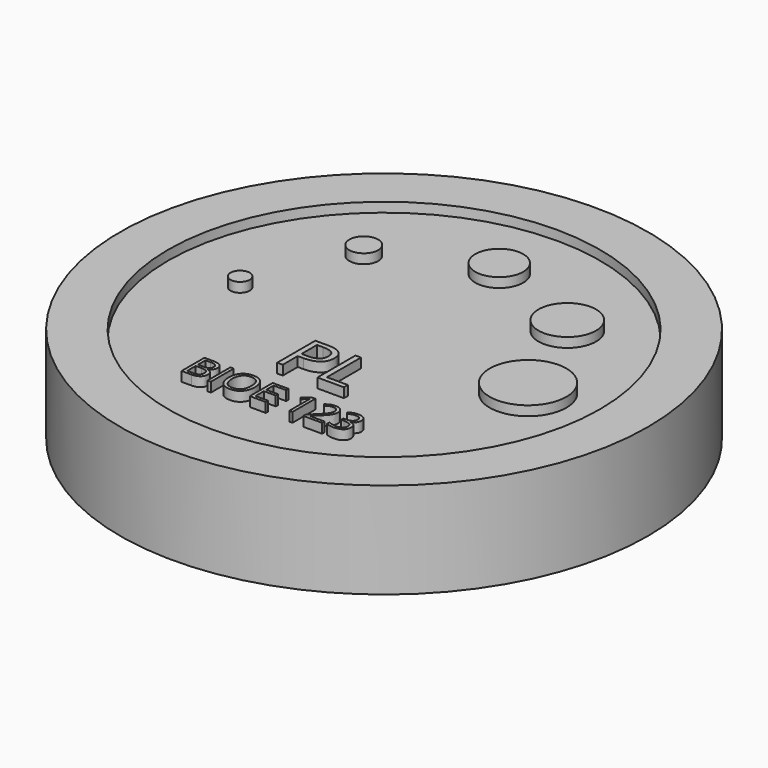
from build123d import *

# Parameters (mm, degrees)
F0_R           = 27.5
F0_R_2         = 22.5
F0_R_3         = 4
F0_R_4         = 3
F0_R_5         = 2.5
F0_R_6         = 1.5
F0_TEXT_SIZE   = 6.9444444444
F0_R_7         = 1
F0_TEXT_SIZE_2 = 4.1666666667
F1_DEPTH       = 10
F0_W           = 0.345703125
F0_H           = 2.974609375
F2_DEPTH       = 3
F4_R           = 22.5
F4_W           = 0.345703125
F4_H           = 2.974609375
F4_R_2         = 1
F4_R_3         = 1.5
F4_R_4         = 3
F4_R_5         = 4
F4_R_6         = 2.5
F5_DEPTH       = 6


# Not quite as in the source:
# - Text() gives the source's letters only with a copy of the font that has no kerning and outlines rounded to 1/6400 em; it was checked with that copy


with BuildPart() as f1:
    # F0 (on Top) → F1 (new body)
    with BuildSketch(Plane.XY):
        Circle(F0_R)
        Circle(F0_R_2, mode=Mode.SUBTRACT)
        with Locations((15, 0)):
            Circle(F0_R_3)
        with Locations((10.6032023465, 10.61)):
            Circle(F0_R_4)
        with Locations((0, 15)):
            Circle(F0_R_5)
        with Locations((-10.6032023465, 10.61)):
            Circle(F0_R_6)
        with Locations((-3.8129340278, -10)):
            Text('PL', F0_TEXT_SIZE, font='Open Sans', text_align=(TextAlign.LEFT, TextAlign.BOTTOM))
        with Locations((-15, 0)):
            Circle(F0_R_7)
        with Locations((-8.7041015625, -16)):
            Text('BIOE 123', F0_TEXT_SIZE_2, font='Open Sans', text_align=(TextAlign.LEFT, TextAlign.BOTTOM))
    extrude(amount=F1_DEPTH)


with BuildPart() as f2:
    # F0 (on Top) → F2 (new body)
    with BuildSketch(Plane.XY):
        Circle(F0_R_2)
        with BuildLine():
            Line((-8.2952473958, -16), (-8.2952473958, -13.025390625))
            Line((-8.2952473958, -13.025390625), (-7.4547526042, -13.025390625))
            add(Edge.make_bspline(
                [(-7.4547526042, -13.025390625), (-6.8629557292, -13.025390625), (-6.5983072917, -13.2024739583)],
                knots=[0, 0, 0, 1, 1, 1], degree=2))
            add(Edge.make_bspline(
                [(-6.5983072917, -13.2024739583), (-6.3336588542, -13.3795572917), (-6.3336588542, -13.76171875)],
                knots=[0, 0, 0, 1, 1, 1], degree=2))
            add(Edge.make_bspline(
                [(-6.3336588542, -13.76171875), (-6.3336588542, -14.0266927083), (-6.4811197917, -14.1985677083)],
                knots=[0, 0, 0, 1, 1, 1], degree=2))
            add(Edge.make_bspline(
                [(-6.4811197917, -14.1985677083), (-6.6285807292, -14.3704427083), (-6.9117838542, -14.4212239583)],
                knots=[0, 0, 0, 1, 1, 1], degree=2))
            Line((-6.9117838542, -14.4212239583), (-6.9117838542, -14.44140625))
            add(Edge.make_bspline(
                [(-6.9117838542, -14.44140625), (-6.2340494792, -14.5572916667), (-6.2340494792, -15.1536458333)],
                knots=[0, 0, 0, 1, 1, 1], degree=2))
            add(Edge.make_bspline(
                [(-6.2340494792, -15.1536458333), (-6.2340494792, -15.5520833333), (-6.5035807292, -15.7760416667)],
                knots=[0, 0, 0, 1, 1, 1], degree=2))
            add(Edge.make_bspline(
                [(-6.5035807292, -15.7760416667), (-6.7731119792, -16), (-7.2574869792, -16)],
                knots=[0, 0, 0, 1, 1, 1], degree=2))
            Line((-7.2574869792, -16), (-8.2952473958, -16))
        make_face(mode=Mode.SUBTRACT)
        with Locations((-5.4225260417, -14.5126953125)):
            Rectangle(F0_W, F0_H, mode=Mode.SUBTRACT)
        with BuildLine():
            add(Edge.make_bspline(
                [(-2.2119140625, -13.3854166667), (-1.8518880208, -13.7923177083), (-1.8518880208, -14.5084635417)],
                knots=[0, 0, 0, 1, 1, 1], degree=2))
            add(Edge.make_bspline(
                [(-1.8518880208, -14.5084635417), (-1.8518880208, -15.22265625), (-2.2132161458, -15.6318359375)],
                knots=[0, 0, 0, 1, 1, 1], degree=2))
            add(Edge.make_bspline(
                [(-2.2132161458, -15.6318359375), (-2.5745442708, -16.041015625), (-3.2171223958, -16.041015625)],
                knots=[0, 0, 0, 1, 1, 1], degree=2))
            add(Edge.make_bspline(
                [(-3.2171223958, -16.041015625), (-3.8740234375, -16.041015625), (-4.2311197917, -15.6389973958)],
                knots=[0, 0, 0, 1, 1, 1], degree=2))
            add(Edge.make_bspline(
                [(-4.2311197917, -15.6389973958), (-4.5882161458, -15.2369791667), (-4.5882161458, -14.5045572917)],
                knots=[0, 0, 0, 1, 1, 1], degree=2))
            add(Edge.make_bspline(
                [(-4.5882161458, -14.5045572917), (-4.5882161458, -13.7779947917), (-4.2301432292, -13.3782552083)],
                knots=[0, 0, 0, 1, 1, 1], degree=2))
            add(Edge.make_bspline(
                [(-4.2301432292, -13.3782552083), (-3.8720703125, -12.978515625), (-3.2132161458, -12.978515625)],
                knots=[0, 0, 0, 1, 1, 1], degree=2))
            add(Edge.make_bspline(
                [(-3.2132161458, -12.978515625), (-2.5719401042, -12.978515625), (-2.2119140625, -13.3854166667)],
                knots=[0, 0, 0, 1, 1, 1], degree=2))
        make_face(mode=Mode.SUBTRACT)
        Polygon((0.4690755208, -15.6907552083), (0.4690755208, -16), (-1.1891276042, -16), (-1.1891276042, -13.025390625), (0.4690755208, -13.025390625), (0.4690755208, -13.3326822917), (-0.8434244792, -13.3326822917), (-0.8434244792, -14.291015625), (0.3896484375, -14.291015625), (0.3896484375, -14.5963541667), (-0.8434244792, -14.5963541667), (-0.8434244792, -15.6907552083), align=None, mode=Mode.SUBTRACT)
        with BuildLine():
            add(Edge.make_bspline(
                [(-1.845703125, -5.0423177083), (0.0119357639, -5.0423177083), (0.0119357639, -6.4865451389)],
                knots=[0, 0, 0, 1, 1, 1], degree=2))
            add(Edge.make_bspline(
                [(0.0119357639, -6.4865451389), (0.0119357639, -7.2395833333), (-0.5018446181, -7.6448567708)],
                knots=[0, 0, 0, 1, 1, 1], degree=2))
            add(Edge.make_bspline(
                [(-0.5018446181, -7.6448567708), (-1.015625, -8.0501302083), (-1.9715711806, -8.0501302083)],
                knots=[0, 0, 0, 1, 1, 1], degree=2))
            Line((-1.9715711806, -8.0501302083), (-2.5553385417, -8.0501302083))
            Line((-2.5553385417, -8.0501302083), (-2.5553385417, -10))
            Line((-2.5553385417, -10), (-3.1315104167, -10))
            Line((-3.1315104167, -10), (-3.1315104167, -5.0423177083))
            Line((-3.1315104167, -5.0423177083), (-1.845703125, -5.0423177083))
        make_face(mode=Mode.SUBTRACT)
        with BuildLine():
            Line((3.2561848958, -13.025390625), (3.2561848958, -16))
            Line((3.2561848958, -16), (2.9267578125, -16))
            Line((2.9267578125, -16), (2.9267578125, -13.8802083333))
            add(Edge.make_bspline(
                [(2.9267578125, -13.8802083333), (2.9267578125, -13.615234375), (2.9430338542, -13.3795572917)],
                knots=[0, 0, 0, 1, 1, 1], degree=2))
            add(Edge.make_bspline(
                [(2.9430338542, -13.3795572917), (2.9007161458, -13.4225260417), (2.84765625, -13.4690755208)],
                knots=[0, 0, 0, 1, 1, 1], degree=2))
            add(Edge.make_bspline(
                [(2.84765625, -13.4690755208), (2.7945963542, -13.515625), (2.3636067708, -13.8658854167)],
                knots=[0, 0, 0, 1, 1, 1], degree=2))
            Line((2.3636067708, -13.8658854167), (2.1845703125, -13.6341145833))
            Line((2.1845703125, -13.6341145833), (2.9716796875, -13.025390625))
            Line((2.9716796875, -13.025390625), (3.2561848958, -13.025390625))
        make_face(mode=Mode.SUBTRACT)
        with BuildLine():
            Line((6.3427734375, -15.6868489583), (6.3427734375, -16))
            Line((6.3427734375, -16), (4.3876953125, -16))
            Line((4.3876953125, -16), (4.3876953125, -15.708984375))
            Line((4.3876953125, -15.708984375), (5.1708984375, -14.921875))
            add(Edge.make_bspline(
                [(5.1708984375, -14.921875), (5.5289713542, -14.5592447917), (5.6429036458, -14.4046223958)],
                knots=[0, 0, 0, 1, 1, 1], degree=2))
            add(Edge.make_bspline(
                [(5.6429036458, -14.4046223958), (5.7568359375, -14.25), (5.8138020833, -14.103515625)],
                knots=[0, 0, 0, 1, 1, 1], degree=2))
            add(Edge.make_bspline(
                [(5.8138020833, -14.103515625), (5.8707682292, -13.95703125), (5.8707682292, -13.7884114583)],
                knots=[0, 0, 0, 1, 1, 1], degree=2))
            add(Edge.make_bspline(
                [(5.8707682292, -13.7884114583), (5.8707682292, -13.5501302083), (5.7262369792, -13.4108072917)],
                knots=[0, 0, 0, 1, 1, 1], degree=2))
            add(Edge.make_bspline(
                [(5.7262369792, -13.4108072917), (5.5817057292, -13.271484375), (5.3251953125, -13.271484375)],
                knots=[0, 0, 0, 1, 1, 1], degree=2))
            add(Edge.make_bspline(
                [(5.3251953125, -13.271484375), (5.1402994792, -13.271484375), (4.9742838542, -13.3326822917)],
                knots=[0, 0, 0, 1, 1, 1], degree=2))
            add(Edge.make_bspline(
                [(4.9742838542, -13.3326822917), (4.8082682292, -13.3938802083), (4.6051432292, -13.5546875)],
                knots=[0, 0, 0, 1, 1, 1], degree=2))
            Line((4.6051432292, -13.5546875), (4.4261067708, -13.3248697917))
            add(Edge.make_bspline(
                [(4.4261067708, -13.3248697917), (4.8369140625, -12.9830729167), (5.3212890625, -12.9830729167)],
                knots=[0, 0, 0, 1, 1, 1], degree=2))
            add(Edge.make_bspline(
                [(5.3212890625, -12.9830729167), (5.7405598958, -12.9830729167), (5.978515625, -13.1975911458)],
                knots=[0, 0, 0, 1, 1, 1], degree=2))
            add(Edge.make_bspline(
                [(5.978515625, -13.1975911458), (6.2164713542, -13.412109375), (6.2164713542, -13.7740885417)],
                knots=[0, 0, 0, 1, 1, 1], degree=2))
            add(Edge.make_bspline(
                [(6.2164713542, -13.7740885417), (6.2164713542, -14.0572916667), (6.0576171875, -14.333984375)],
                knots=[0, 0, 0, 1, 1, 1], degree=2))
            add(Edge.make_bspline(
                [(6.0576171875, -14.333984375), (5.8987630208, -14.6106770833), (5.4638671875, -15.0338541667)],
                knots=[0, 0, 0, 1, 1, 1], degree=2))
            Line((5.4638671875, -15.0338541667), (4.8128255208, -15.6705729167))
            Line((4.8128255208, -15.6705729167), (4.8128255208, -15.6868489583))
            Line((4.8128255208, -15.6868489583), (6.3427734375, -15.6868489583))
        make_face(mode=Mode.SUBTRACT)
        with BuildLine():
            add(Edge.make_bspline(
                [(8.3727213542, -13.1813151042), (8.6129557292, -13.3795572917), (8.6129557292, -13.7252604167)],
                knots=[0, 0, 0, 1, 1, 1], degree=2))
            add(Edge.make_bspline(
                [(8.6129557292, -13.7252604167), (8.6129557292, -14.0104166667), (8.453125, -14.19140625)],
                knots=[0, 0, 0, 1, 1, 1], degree=2))
            add(Edge.make_bspline(
                [(8.453125, -14.19140625), (8.2932942708, -14.3723958333), (8.0003255208, -14.43359375)],
                knots=[0, 0, 0, 1, 1, 1], degree=2))
            Line((8.0003255208, -14.43359375), (8.0003255208, -14.4498697917))
            add(Edge.make_bspline(
                [(8.0003255208, -14.4498697917), (8.3583984375, -14.494140625), (8.53125, -14.6774088542)],
                knots=[0, 0, 0, 1, 1, 1], degree=2))
            add(Edge.make_bspline(
                [(8.53125, -14.6774088542), (8.7041015625, -14.8606770833), (8.7041015625, -15.1575520833)],
                knots=[0, 0, 0, 1, 1, 1], degree=2))
            add(Edge.make_bspline(
                [(8.7041015625, -15.1575520833), (8.7041015625, -15.5826822917), (8.4091796875, -15.8118489583)],
                knots=[0, 0, 0, 1, 1, 1], degree=2))
            add(Edge.make_bspline(
                [(8.4091796875, -15.8118489583), (8.1142578125, -16.041015625), (7.5712890625, -16.041015625)],
                knots=[0, 0, 0, 1, 1, 1], degree=2))
            add(Edge.make_bspline(
                [(7.5712890625, -16.041015625), (7.3349609375, -16.041015625), (7.138671875, -16.0052083333)],
                knots=[0, 0, 0, 1, 1, 1], degree=2))
            add(Edge.make_bspline(
                [(7.138671875, -16.0052083333), (6.9423828125, -15.9694010417), (6.7574869792, -15.8802083333)],
                knots=[0, 0, 0, 1, 1, 1], degree=2))
            Line((6.7574869792, -15.8802083333), (6.7574869792, -15.55859375))
            add(Edge.make_bspline(
                [(6.7574869792, -15.55859375), (6.9508463542, -15.654296875), (7.1695963542, -15.7041015625)],
                knots=[0, 0, 0, 1, 1, 1], degree=2))
            add(Edge.make_bspline(
                [(7.1695963542, -15.7041015625), (7.3883463542, -15.75390625), (7.5836588542, -15.75390625)],
                knots=[0, 0, 0, 1, 1, 1], degree=2))
            add(Edge.make_bspline(
                [(7.5836588542, -15.75390625), (8.3544921875, -15.75390625), (8.3544921875, -15.1497395833)],
                knots=[0, 0, 0, 1, 1, 1], degree=2))
            add(Edge.make_bspline(
                [(8.3544921875, -15.1497395833), (8.3544921875, -14.6080729167), (7.5042317708, -14.6080729167)],
                knots=[0, 0, 0, 1, 1, 1], degree=2))
            Line((7.5042317708, -14.6080729167), (7.2112630208, -14.6080729167))
            Line((7.2112630208, -14.6080729167), (7.2112630208, -14.3177083333))
            Line((7.2112630208, -14.3177083333), (7.5081380208, -14.3177083333))
            add(Edge.make_bspline(
                [(7.5081380208, -14.3177083333), (7.8557942708, -14.3177083333), (8.0592447917, -14.1640625)],
                knots=[0, 0, 0, 1, 1, 1], degree=2))
            add(Edge.make_bspline(
                [(8.0592447917, -14.1640625), (8.2626953125, -14.0104166667), (8.2626953125, -13.7376302083)],
                knots=[0, 0, 0, 1, 1, 1], degree=2))
            add(Edge.make_bspline(
                [(8.2626953125, -13.7376302083), (8.2626953125, -13.5201822917), (8.11328125, -13.3958333333)],
                knots=[0, 0, 0, 1, 1, 1], degree=2))
            add(Edge.make_bspline(
                [(8.11328125, -13.3958333333), (7.9638671875, -13.271484375), (7.7073567708, -13.271484375)],
                knots=[0, 0, 0, 1, 1, 1], degree=2))
            add(Edge.make_bspline(
                [(7.7073567708, -13.271484375), (7.5120442708, -13.271484375), (7.3391927083, -13.3245442708)],
                knots=[0, 0, 0, 1, 1, 1], degree=2))
            add(Edge.make_bspline(
                [(7.3391927083, -13.3245442708), (7.1663411458, -13.3776041667), (6.9443359375, -13.5201822917)],
                knots=[0, 0, 0, 1, 1, 1], degree=2))
            Line((6.9443359375, -13.5201822917), (6.7737630208, -13.2923177083))
            add(Edge.make_bspline(
                [(6.7737630208, -13.2923177083), (6.9567057292, -13.1477864583), (7.1956380208, -13.0654296875)],
                knots=[0, 0, 0, 1, 1, 1], degree=2))
            add(Edge.make_bspline(
                [(7.1956380208, -13.0654296875), (7.4345703125, -12.9830729167), (7.6995442708, -12.9830729167)],
                knots=[0, 0, 0, 1, 1, 1], degree=2))
            add(Edge.make_bspline(
                [(7.6995442708, -12.9830729167), (8.1324869792, -12.9830729167), (8.3727213542, -13.1813151042)],
                knots=[0, 0, 0, 1, 1, 1], degree=2))
        make_face(mode=Mode.SUBTRACT)
        Polygon((3.8129340278, -10), (1.0492621528, -10), (1.0492621528, -5.0423177083), (1.6254340278, -5.0423177083), (1.6254340278, -9.4780815972), (3.8129340278, -9.4780815972), align=None, mode=Mode.SUBTRACT)
        with Locations((-15, 0)):
            Circle(F0_R_7, mode=Mode.SUBTRACT)
        with Locations((-10.6032023465, 10.61)):
            Circle(F0_R_6, mode=Mode.SUBTRACT)
        with Locations((10.6032023465, 10.61)):
            Circle(F0_R_4, mode=Mode.SUBTRACT)
        with Locations((15, 0)):
            Circle(F0_R_3, mode=Mode.SUBTRACT)
        with Locations((0, 15)):
            Circle(F0_R_5, mode=Mode.SUBTRACT)
    extrude(amount=F2_DEPTH)


with BuildPart() as f2b:
    # F0 (on Top) → F2, piece 2 (new body)
    with BuildSketch(Plane.XY):
        with BuildLine():
            Line((-2.5553385417, -5.5414496528), (-2.5553385417, -7.5553385417))
            Line((-2.5553385417, -7.5553385417), (-2.0355902778, -7.5553385417))
            add(Edge.make_bspline(
                [(-2.0355902778, -7.5553385417), (-1.26953125, -7.5553385417), (-0.9271918403, -7.3079427083)],
                knots=[0, 0, 0, 1, 1, 1], degree=2))
            add(Edge.make_bspline(
                [(-0.9271918403, -7.3079427083), (-0.5848524306, -7.060546875), (-0.5848524306, -6.513671875)],
                knots=[0, 0, 0, 1, 1, 1], degree=2))
            add(Edge.make_bspline(
                [(-0.5848524306, -6.513671875), (-0.5848524306, -6.0221354167), (-0.9071180556, -5.7817925347)],
                knots=[0, 0, 0, 1, 1, 1], degree=2))
            add(Edge.make_bspline(
                [(-0.9071180556, -5.7817925347), (-1.2293836806, -5.5414496528), (-1.9108072917, -5.5414496528)],
                knots=[0, 0, 0, 1, 1, 1], degree=2))
            Line((-1.9108072917, -5.5414496528), (-2.5553385417, -5.5414496528))
        make_face()
    extrude(amount=F2_DEPTH)


with BuildPart() as f2c:
    # F0 (on Top) → F2, piece 3 (new body)
    with BuildSketch(Plane.XY):
        with BuildLine():
            add(Edge.make_bspline(
                [(-3.96484375, -13.6002604167), (-4.2223307292, -13.9127604167), (-4.2223307292, -14.5084635417)],
                knots=[0, 0, 0, 1, 1, 1], degree=2))
            add(Edge.make_bspline(
                [(-4.2223307292, -14.5084635417), (-4.2223307292, -15.1126302083), (-3.96484375, -15.4251302083)],
                knots=[0, 0, 0, 1, 1, 1], degree=2))
            add(Edge.make_bspline(
                [(-3.96484375, -15.4251302083), (-3.7073567708, -15.7376302083), (-3.2171223958, -15.7376302083)],
                knots=[0, 0, 0, 1, 1, 1], degree=2))
            add(Edge.make_bspline(
                [(-3.2171223958, -15.7376302083), (-2.7229817708, -15.7376302083), (-2.470703125, -15.4264322917)],
                knots=[0, 0, 0, 1, 1, 1], degree=2))
            add(Edge.make_bspline(
                [(-2.470703125, -15.4264322917), (-2.2184244792, -15.115234375), (-2.2184244792, -14.5084635417)],
                knots=[0, 0, 0, 1, 1, 1], degree=2))
            add(Edge.make_bspline(
                [(-2.2184244792, -14.5084635417), (-2.2184244792, -13.908203125), (-2.4697265625, -13.5979817708)],
                knots=[0, 0, 0, 1, 1, 1], degree=2))
            add(Edge.make_bspline(
                [(-2.4697265625, -13.5979817708), (-2.7210286458, -13.2877604167), (-3.2132161458, -13.2877604167)],
                knots=[0, 0, 0, 1, 1, 1], degree=2))
            add(Edge.make_bspline(
                [(-3.2132161458, -13.2877604167), (-3.7073567708, -13.2877604167), (-3.96484375, -13.6002604167)],
                knots=[0, 0, 0, 1, 1, 1], degree=2))
        make_face()
    extrude(amount=F2_DEPTH)


with BuildPart() as f2d:
    # F0 (on Top) → F2, piece 4 (new body)
    with BuildSketch(Plane.XY):
        with BuildLine():
            Line((-7.9495442708, -13.3248697917), (-7.9495442708, -14.298828125))
            Line((-7.9495442708, -14.298828125), (-7.3798828125, -14.298828125))
            add(Edge.make_bspline(
                [(-7.3798828125, -14.298828125), (-7.0133463542, -14.298828125), (-6.8525390625, -14.1839192708)],
                knots=[0, 0, 0, 1, 1, 1], degree=2))
            add(Edge.make_bspline(
                [(-6.8525390625, -14.1839192708), (-6.6917317708, -14.0690104167), (-6.6917317708, -13.796875)],
                knots=[0, 0, 0, 1, 1, 1], degree=2))
            add(Edge.make_bspline(
                [(-6.6917317708, -13.796875), (-6.6917317708, -13.5462239583), (-6.8707682292, -13.435546875)],
                knots=[0, 0, 0, 1, 1, 1], degree=2))
            add(Edge.make_bspline(
                [(-6.8707682292, -13.435546875), (-7.0498046875, -13.3248697917), (-7.4404296875, -13.3248697917)],
                knots=[0, 0, 0, 1, 1, 1], degree=2))
            Line((-7.4404296875, -13.3248697917), (-7.9495442708, -13.3248697917))
        make_face()
    extrude(amount=F2_DEPTH)


with BuildPart() as f2e:
    # F0 (on Top) → F2, piece 5 (new body)
    with BuildSketch(Plane.XY):
        with BuildLine():
            Line((-7.3570963542, -14.591796875), (-7.9495442708, -14.591796875))
            Line((-7.9495442708, -14.591796875), (-7.9495442708, -15.705078125))
            Line((-7.9495442708, -15.705078125), (-7.3284505208, -15.705078125))
            add(Edge.make_bspline(
                [(-7.3284505208, -15.705078125), (-6.9684244792, -15.705078125), (-6.7864583333, -15.5657552083)],
                knots=[0, 0, 0, 1, 1, 1], degree=2))
            add(Edge.make_bspline(
                [(-6.7864583333, -15.5657552083), (-6.6044921875, -15.4264322917), (-6.6044921875, -15.12890625)],
                knots=[0, 0, 0, 1, 1, 1], degree=2))
            add(Edge.make_bspline(
                [(-6.6044921875, -15.12890625), (-6.6044921875, -14.8522135417), (-6.7906901042, -14.7220052083)],
                knots=[0, 0, 0, 1, 1, 1], degree=2))
            add(Edge.make_bspline(
                [(-6.7906901042, -14.7220052083), (-6.9768880208, -14.591796875), (-7.3570963542, -14.591796875)],
                knots=[0, 0, 0, 1, 1, 1], degree=2))
        make_face()
    extrude(amount=F2_DEPTH)


with BuildPart() as f5:
    # F4 (on offset) → F5 (new body)
    with BuildSketch(Plane.XY.offset(3)):
        Circle(F4_R)
        with BuildLine():
            Line((-8.2952473958, -16), (-8.2952473958, -13.025390625))
            Line((-8.2952473958, -13.025390625), (-7.4547526042, -13.025390625))
            add(Edge.make_bspline(
                [(-7.4547526042, -13.025390625), (-6.8629557292, -13.025390625), (-6.5983072917, -13.2024739583)],
                knots=[0, 0, 0, 1, 1, 1], degree=2))
            add(Edge.make_bspline(
                [(-6.5983072917, -13.2024739583), (-6.3336588542, -13.3795572917), (-6.3336588542, -13.76171875)],
                knots=[0, 0, 0, 1, 1, 1], degree=2))
            add(Edge.make_bspline(
                [(-6.3336588542, -13.76171875), (-6.3336588542, -14.0266927083), (-6.4811197917, -14.1985677083)],
                knots=[0, 0, 0, 1, 1, 1], degree=2))
            add(Edge.make_bspline(
                [(-6.4811197917, -14.1985677083), (-6.6285807292, -14.3704427083), (-6.9117838542, -14.4212239583)],
                knots=[0, 0, 0, 1, 1, 1], degree=2))
            Line((-6.9117838542, -14.4212239583), (-6.9117838542, -14.44140625))
            add(Edge.make_bspline(
                [(-6.9117838542, -14.44140625), (-6.2340494792, -14.5572916667), (-6.2340494792, -15.1536458333)],
                knots=[0, 0, 0, 1, 1, 1], degree=2))
            add(Edge.make_bspline(
                [(-6.2340494792, -15.1536458333), (-6.2340494792, -15.5520833333), (-6.5035807292, -15.7760416667)],
                knots=[0, 0, 0, 1, 1, 1], degree=2))
            add(Edge.make_bspline(
                [(-6.5035807292, -15.7760416667), (-6.7731119792, -16), (-7.2574869792, -16)],
                knots=[0, 0, 0, 1, 1, 1], degree=2))
            Line((-7.2574869792, -16), (-8.2952473958, -16))
        make_face(mode=Mode.SUBTRACT)
        with Locations((-5.4225260417, -14.5126953125)):
            Rectangle(F4_W, F4_H, mode=Mode.SUBTRACT)
        with BuildLine():
            add(Edge.make_bspline(
                [(-2.2119140625, -13.3854166667), (-1.8518880208, -13.7923177083), (-1.8518880208, -14.5084635417)],
                knots=[0, 0, 0, 1, 1, 1], degree=2))
            add(Edge.make_bspline(
                [(-1.8518880208, -14.5084635417), (-1.8518880208, -15.22265625), (-2.2132161458, -15.6318359375)],
                knots=[0, 0, 0, 1, 1, 1], degree=2))
            add(Edge.make_bspline(
                [(-2.2132161458, -15.6318359375), (-2.5745442708, -16.041015625), (-3.2171223958, -16.041015625)],
                knots=[0, 0, 0, 1, 1, 1], degree=2))
            add(Edge.make_bspline(
                [(-3.2171223958, -16.041015625), (-3.8740234375, -16.041015625), (-4.2311197917, -15.6389973958)],
                knots=[0, 0, 0, 1, 1, 1], degree=2))
            add(Edge.make_bspline(
                [(-4.2311197917, -15.6389973958), (-4.5882161458, -15.2369791667), (-4.5882161458, -14.5045572917)],
                knots=[0, 0, 0, 1, 1, 1], degree=2))
            add(Edge.make_bspline(
                [(-4.5882161458, -14.5045572917), (-4.5882161458, -13.7779947917), (-4.2301432292, -13.3782552083)],
                knots=[0, 0, 0, 1, 1, 1], degree=2))
            add(Edge.make_bspline(
                [(-4.2301432292, -13.3782552083), (-3.8720703125, -12.978515625), (-3.2132161458, -12.978515625)],
                knots=[0, 0, 0, 1, 1, 1], degree=2))
            add(Edge.make_bspline(
                [(-3.2132161458, -12.978515625), (-2.5719401042, -12.978515625), (-2.2119140625, -13.3854166667)],
                knots=[0, 0, 0, 1, 1, 1], degree=2))
        make_face(mode=Mode.SUBTRACT)
        Polygon((0.4690755208, -15.6907552083), (0.4690755208, -16), (-1.1891276042, -16), (-1.1891276042, -13.025390625), (0.4690755208, -13.025390625), (0.4690755208, -13.3326822917), (-0.8434244792, -13.3326822917), (-0.8434244792, -14.291015625), (0.3896484375, -14.291015625), (0.3896484375, -14.5963541667), (-0.8434244792, -14.5963541667), (-0.8434244792, -15.6907552083), align=None, mode=Mode.SUBTRACT)
        with BuildLine():
            add(Edge.make_bspline(
                [(-1.845703125, -5.0423177083), (0.0119357639, -5.0423177083), (0.0119357639, -6.4865451389)],
                knots=[0, 0, 0, 1, 1, 1], degree=2))
            add(Edge.make_bspline(
                [(0.0119357639, -6.4865451389), (0.0119357639, -7.2395833333), (-0.5018446181, -7.6448567708)],
                knots=[0, 0, 0, 1, 1, 1], degree=2))
            add(Edge.make_bspline(
                [(-0.5018446181, -7.6448567708), (-1.015625, -8.0501302083), (-1.9715711806, -8.0501302083)],
                knots=[0, 0, 0, 1, 1, 1], degree=2))
            Line((-1.9715711806, -8.0501302083), (-2.5553385417, -8.0501302083))
            Line((-2.5553385417, -8.0501302083), (-2.5553385417, -10))
            Line((-2.5553385417, -10), (-3.1315104167, -10))
            Line((-3.1315104167, -10), (-3.1315104167, -5.0423177083))
            Line((-3.1315104167, -5.0423177083), (-1.845703125, -5.0423177083))
        make_face(mode=Mode.SUBTRACT)
        with BuildLine():
            Line((3.2561848958, -13.025390625), (3.2561848958, -16))
            Line((3.2561848958, -16), (2.9267578125, -16))
            Line((2.9267578125, -16), (2.9267578125, -13.8802083333))
            add(Edge.make_bspline(
                [(2.9267578125, -13.8802083333), (2.9267578125, -13.615234375), (2.9430338542, -13.3795572917)],
                knots=[0, 0, 0, 1, 1, 1], degree=2))
            add(Edge.make_bspline(
                [(2.9430338542, -13.3795572917), (2.9007161458, -13.4225260417), (2.84765625, -13.4690755208)],
                knots=[0, 0, 0, 1, 1, 1], degree=2))
            add(Edge.make_bspline(
                [(2.84765625, -13.4690755208), (2.7945963542, -13.515625), (2.3636067708, -13.8658854167)],
                knots=[0, 0, 0, 1, 1, 1], degree=2))
            Line((2.3636067708, -13.8658854167), (2.1845703125, -13.6341145833))
            Line((2.1845703125, -13.6341145833), (2.9716796875, -13.025390625))
            Line((2.9716796875, -13.025390625), (3.2561848958, -13.025390625))
        make_face(mode=Mode.SUBTRACT)
        with BuildLine():
            Line((6.3427734375, -15.6868489583), (6.3427734375, -16))
            Line((6.3427734375, -16), (4.3876953125, -16))
            Line((4.3876953125, -16), (4.3876953125, -15.708984375))
            Line((4.3876953125, -15.708984375), (5.1708984375, -14.921875))
            add(Edge.make_bspline(
                [(5.1708984375, -14.921875), (5.5289713542, -14.5592447917), (5.6429036458, -14.4046223958)],
                knots=[0, 0, 0, 1, 1, 1], degree=2))
            add(Edge.make_bspline(
                [(5.6429036458, -14.4046223958), (5.7568359375, -14.25), (5.8138020833, -14.103515625)],
                knots=[0, 0, 0, 1, 1, 1], degree=2))
            add(Edge.make_bspline(
                [(5.8138020833, -14.103515625), (5.8707682292, -13.95703125), (5.8707682292, -13.7884114583)],
                knots=[0, 0, 0, 1, 1, 1], degree=2))
            add(Edge.make_bspline(
                [(5.8707682292, -13.7884114583), (5.8707682292, -13.5501302083), (5.7262369792, -13.4108072917)],
                knots=[0, 0, 0, 1, 1, 1], degree=2))
            add(Edge.make_bspline(
                [(5.7262369792, -13.4108072917), (5.5817057292, -13.271484375), (5.3251953125, -13.271484375)],
                knots=[0, 0, 0, 1, 1, 1], degree=2))
            add(Edge.make_bspline(
                [(5.3251953125, -13.271484375), (5.1402994792, -13.271484375), (4.9742838542, -13.3326822917)],
                knots=[0, 0, 0, 1, 1, 1], degree=2))
            add(Edge.make_bspline(
                [(4.9742838542, -13.3326822917), (4.8082682292, -13.3938802083), (4.6051432292, -13.5546875)],
                knots=[0, 0, 0, 1, 1, 1], degree=2))
            Line((4.6051432292, -13.5546875), (4.4261067708, -13.3248697917))
            add(Edge.make_bspline(
                [(4.4261067708, -13.3248697917), (4.8369140625, -12.9830729167), (5.3212890625, -12.9830729167)],
                knots=[0, 0, 0, 1, 1, 1], degree=2))
            add(Edge.make_bspline(
                [(5.3212890625, -12.9830729167), (5.7405598958, -12.9830729167), (5.978515625, -13.1975911458)],
                knots=[0, 0, 0, 1, 1, 1], degree=2))
            add(Edge.make_bspline(
                [(5.978515625, -13.1975911458), (6.2164713542, -13.412109375), (6.2164713542, -13.7740885417)],
                knots=[0, 0, 0, 1, 1, 1], degree=2))
            add(Edge.make_bspline(
                [(6.2164713542, -13.7740885417), (6.2164713542, -14.0572916667), (6.0576171875, -14.333984375)],
                knots=[0, 0, 0, 1, 1, 1], degree=2))
            add(Edge.make_bspline(
                [(6.0576171875, -14.333984375), (5.8987630208, -14.6106770833), (5.4638671875, -15.0338541667)],
                knots=[0, 0, 0, 1, 1, 1], degree=2))
            Line((5.4638671875, -15.0338541667), (4.8128255208, -15.6705729167))
            Line((4.8128255208, -15.6705729167), (4.8128255208, -15.6868489583))
            Line((4.8128255208, -15.6868489583), (6.3427734375, -15.6868489583))
        make_face(mode=Mode.SUBTRACT)
        with BuildLine():
            add(Edge.make_bspline(
                [(8.3727213542, -13.1813151042), (8.6129557292, -13.3795572917), (8.6129557292, -13.7252604167)],
                knots=[0, 0, 0, 1, 1, 1], degree=2))
            add(Edge.make_bspline(
                [(8.6129557292, -13.7252604167), (8.6129557292, -14.0104166667), (8.453125, -14.19140625)],
                knots=[0, 0, 0, 1, 1, 1], degree=2))
            add(Edge.make_bspline(
                [(8.453125, -14.19140625), (8.2932942708, -14.3723958333), (8.0003255208, -14.43359375)],
                knots=[0, 0, 0, 1, 1, 1], degree=2))
            Line((8.0003255208, -14.43359375), (8.0003255208, -14.4498697917))
            add(Edge.make_bspline(
                [(8.0003255208, -14.4498697917), (8.3583984375, -14.494140625), (8.53125, -14.6774088542)],
                knots=[0, 0, 0, 1, 1, 1], degree=2))
            add(Edge.make_bspline(
                [(8.53125, -14.6774088542), (8.7041015625, -14.8606770833), (8.7041015625, -15.1575520833)],
                knots=[0, 0, 0, 1, 1, 1], degree=2))
            add(Edge.make_bspline(
                [(8.7041015625, -15.1575520833), (8.7041015625, -15.5826822917), (8.4091796875, -15.8118489583)],
                knots=[0, 0, 0, 1, 1, 1], degree=2))
            add(Edge.make_bspline(
                [(8.4091796875, -15.8118489583), (8.1142578125, -16.041015625), (7.5712890625, -16.041015625)],
                knots=[0, 0, 0, 1, 1, 1], degree=2))
            add(Edge.make_bspline(
                [(7.5712890625, -16.041015625), (7.3349609375, -16.041015625), (7.138671875, -16.0052083333)],
                knots=[0, 0, 0, 1, 1, 1], degree=2))
            add(Edge.make_bspline(
                [(7.138671875, -16.0052083333), (6.9423828125, -15.9694010417), (6.7574869792, -15.8802083333)],
                knots=[0, 0, 0, 1, 1, 1], degree=2))
            Line((6.7574869792, -15.8802083333), (6.7574869792, -15.55859375))
            add(Edge.make_bspline(
                [(6.7574869792, -15.55859375), (6.9508463542, -15.654296875), (7.1695963542, -15.7041015625)],
                knots=[0, 0, 0, 1, 1, 1], degree=2))
            add(Edge.make_bspline(
                [(7.1695963542, -15.7041015625), (7.3883463542, -15.75390625), (7.5836588542, -15.75390625)],
                knots=[0, 0, 0, 1, 1, 1], degree=2))
            add(Edge.make_bspline(
                [(7.5836588542, -15.75390625), (8.3544921875, -15.75390625), (8.3544921875, -15.1497395833)],
                knots=[0, 0, 0, 1, 1, 1], degree=2))
            add(Edge.make_bspline(
                [(8.3544921875, -15.1497395833), (8.3544921875, -14.6080729167), (7.5042317708, -14.6080729167)],
                knots=[0, 0, 0, 1, 1, 1], degree=2))
            Line((7.5042317708, -14.6080729167), (7.2112630208, -14.6080729167))
            Line((7.2112630208, -14.6080729167), (7.2112630208, -14.3177083333))
            Line((7.2112630208, -14.3177083333), (7.5081380208, -14.3177083333))
            add(Edge.make_bspline(
                [(7.5081380208, -14.3177083333), (7.8557942708, -14.3177083333), (8.0592447917, -14.1640625)],
                knots=[0, 0, 0, 1, 1, 1], degree=2))
            add(Edge.make_bspline(
                [(8.0592447917, -14.1640625), (8.2626953125, -14.0104166667), (8.2626953125, -13.7376302083)],
                knots=[0, 0, 0, 1, 1, 1], degree=2))
            add(Edge.make_bspline(
                [(8.2626953125, -13.7376302083), (8.2626953125, -13.5201822917), (8.11328125, -13.3958333333)],
                knots=[0, 0, 0, 1, 1, 1], degree=2))
            add(Edge.make_bspline(
                [(8.11328125, -13.3958333333), (7.9638671875, -13.271484375), (7.7073567708, -13.271484375)],
                knots=[0, 0, 0, 1, 1, 1], degree=2))
            add(Edge.make_bspline(
                [(7.7073567708, -13.271484375), (7.5120442708, -13.271484375), (7.3391927083, -13.3245442708)],
                knots=[0, 0, 0, 1, 1, 1], degree=2))
            add(Edge.make_bspline(
                [(7.3391927083, -13.3245442708), (7.1663411458, -13.3776041667), (6.9443359375, -13.5201822917)],
                knots=[0, 0, 0, 1, 1, 1], degree=2))
            Line((6.9443359375, -13.5201822917), (6.7737630208, -13.2923177083))
            add(Edge.make_bspline(
                [(6.7737630208, -13.2923177083), (6.9567057292, -13.1477864583), (7.1956380208, -13.0654296875)],
                knots=[0, 0, 0, 1, 1, 1], degree=2))
            add(Edge.make_bspline(
                [(7.1956380208, -13.0654296875), (7.4345703125, -12.9830729167), (7.6995442708, -12.9830729167)],
                knots=[0, 0, 0, 1, 1, 1], degree=2))
            add(Edge.make_bspline(
                [(7.6995442708, -12.9830729167), (8.1324869792, -12.9830729167), (8.3727213542, -13.1813151042)],
                knots=[0, 0, 0, 1, 1, 1], degree=2))
        make_face(mode=Mode.SUBTRACT)
        Polygon((3.8129340278, -10), (1.0492621528, -10), (1.0492621528, -5.0423177083), (1.6254340278, -5.0423177083), (1.6254340278, -9.4780815972), (3.8129340278, -9.4780815972), align=None, mode=Mode.SUBTRACT)
        with Locations((-15, 0)):
            Circle(F4_R_2, mode=Mode.SUBTRACT)
        with Locations((-10.6032023465, 10.61)):
            Circle(F4_R_3, mode=Mode.SUBTRACT)
        with Locations((10.6032023465, 10.61)):
            Circle(F4_R_4, mode=Mode.SUBTRACT)
        with Locations((15, 0)):
            Circle(F4_R_5, mode=Mode.SUBTRACT)
        with Locations((0, 15)):
            Circle(F4_R_6, mode=Mode.SUBTRACT)
    extrude(amount=F5_DEPTH)


solid = Compound([f1.part, f2.part, f2b.part, f2c.part, f2d.part, f2e.part, f5.part])
